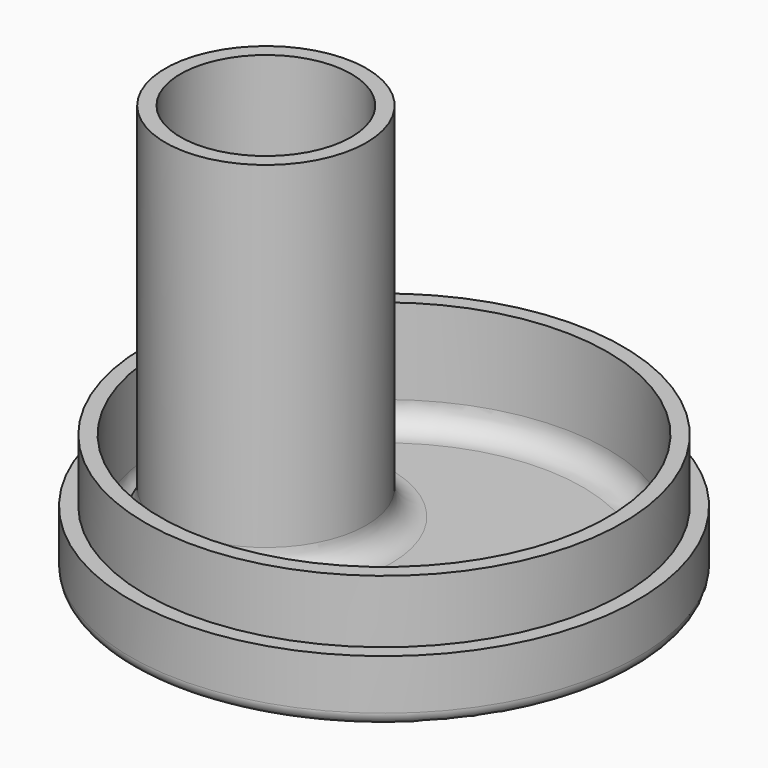
from build123d import *

# Parameters (mm, degrees)
F2_R        = 8
F2_R_2      = 6.8
F3_DEPTH    = 30
F4_R        = 6.7244244579
F5_DEPTH    = 2.5
F6_R        = 1
F7_S7_R     = 8
F7_T8_DEPTH = 29


# Not quite as in the source:
# - a fillet or chamfer that OpenCascade refuses, or shapes differently, is made with other operations: its cross-section is extruded or revolved along the edge and cut away or added


with BuildPart() as f1:
    # F0 (on Front) → F1 (revolve)
    with BuildSketch(Plane.XZ):
        Polygon((-20.2, 0), (0, 0), (0, 1.2), (-17.8, 1.2), (-17.8, 10), (-19, 10), (-19, 5), (-20.2, 5), align=None)
    revolve(axis=Axis((0, 0, 6.5113101155), (0, 0, -1)))

    # F2 (on Top) → F3 (join)
    with BuildSketch(Plane.XY):
        with Locations((-9.4, 0)):
            Circle(F2_R)
        with Locations((-9.4, 0)):
            Circle(F2_R_2, mode=Mode.SUBTRACT)
    extrude(amount=F3_DEPTH)

    # F4 (on Top) → F5 (cut, symmetric)
    with BuildSketch(Plane.XY):
        with Locations((-9.4230027523, -0.008787398)):
            Circle(F4_R)
    extrude(amount=F5_DEPTH, both=True, mode=Mode.SUBTRACT)

    # F6
    f6_edges = [f1.edges().sort_by_distance(p)[0] for p in [
        (20.2, 0, 0),
        (-16.147427, -0.008787, 0),
    ]]
    fillet(f6_edges, radius=F6_R)

    # F7: fillet of radius 2 on 2 edges, made by hand

    # F7_s1 → F7_t2 (revolve)
    with BuildSketch(Plane.XZ):
        with BuildLine():
            ThreePointArc((-1.4, 3.2), (-0.8142135624, 1.7857864376), (0.6, 1.2))
            Line((0.6, 1.2), (-1.4, 1.2))
            Line((-1.4, 1.2), (-1.4, 3.2))
        make_face()
    revolve(axis=Axis((-9.4, 0, 1.2), (0, 0, -1)))


with BuildPart() as f7_tool4:
    # F7_s5 → F7_t6 (revolve)
    with BuildSketch(Plane.XZ):
        with BuildLine():
            ThreePointArc((-17.8, 3.2), (-17.2142135624, 1.7857864376), (-15.8, 1.2))
            Line((-15.8, 1.2), (-17.8, 1.2))
            Line((-17.8, 1.2), (-17.8, 3.2))
        make_face()
    revolve(axis=Axis((0, 0, 1.2), (0, 0, -1)))

    # F7_s7 → F7_t8 (cut, symmetric)
    with BuildSketch(Plane.XY.offset(2.2)):
        with Locations((-9.4, 0)):
            Circle(F7_S7_R)
    extrude(amount=F7_T8_DEPTH, both=True, mode=Mode.SUBTRACT)


with BuildPart() as f1_1:
    add(f1.part)

    # F7_t3: union F7_tool4
    add(f7_tool4.part)


solid = f1_1.part
